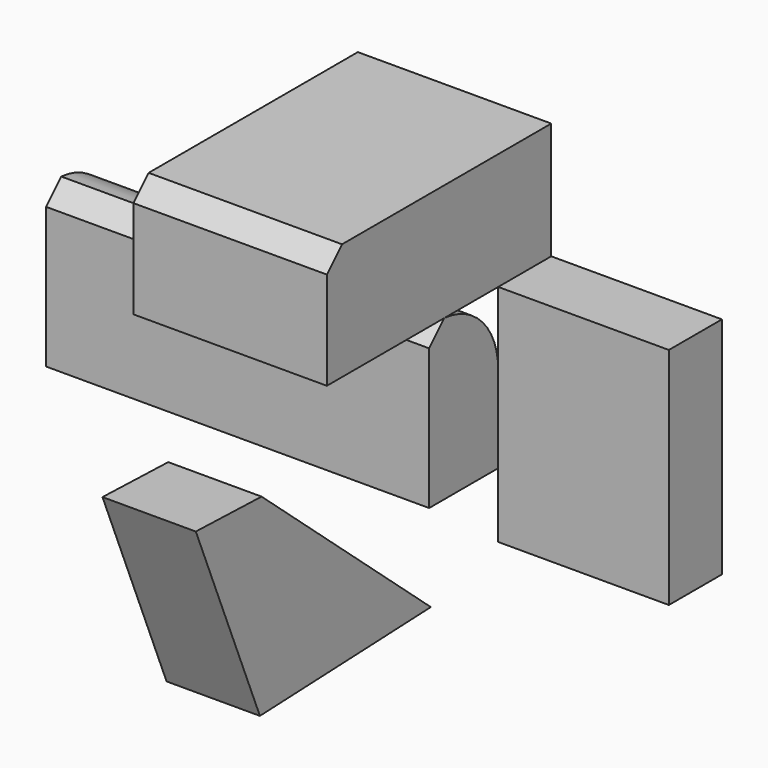
from build123d import *

# Parameters (mm, degrees)
F0_W        = 23.1258124113
F0_H        = 42.7482295781
F1_DEPTH    = 102.616
F2_DEPTH    = 51.816
F3_DEPTH    = 45.72
F4_SIZE     = 5.08
F4_2_SIZE   = 5.08
F5_T1_DEPTH = 200.4123170871
F7_DEPTH    = 12.5


# Not quite as in the source:
# - a fillet or chamfer that OpenCascade refuses, or shapes differently, is made with other operations: its cross-section is extruded or revolved along the edge and cut away or added
# - a feature of the source that left no trace in its solid (it failed there, or was rolled back) is left out


with BuildPart() as f1:
    # F0 (on Right) → F1 (new body)
    with BuildSketch(Plane.YZ):
        with Locations((59.9930435419, 8.5665853694)):
            Rectangle(F0_W, F0_H)
    extrude(amount=-F1_DEPTH)

    # F4
    f4_edges = [f1.edges().sort_by_distance(p)[0] for p in [
        (-51.308, 48.430137, 29.9407),
    ]]
    chamfer(f4_edges, length=F4_SIZE)

    # F5: fillet of radius 19.622727835 on 1 edges, made by hand

    # F5_s2 → F5_t1 (cut)
    with BuildSketch(Plane.YZ.offset(-151.5141585435)):
        with BuildLine():
            ThreePointArc((53.5101373363, 29.9407001585), (66.355337393, 23.687601957), (71.5559497476, 10.3814367411))
            Line((71.5559497476, 10.3814367411), (71.5559497476, 29.9407001585))
            Line((71.5559497476, 29.9407001585), (53.5101373363, 29.9407001585))
        make_face()
    extrude(amount=F5_T1_DEPTH, mode=Mode.SUBTRACT)


with BuildPart() as f2:
    # F0 (on Right) → F2 (new body)
    with BuildSketch(Plane.YZ):
        Polygon((89.3192514777, 29.9407001585), (89.3192514777, 61.2500272691), (14.1880903393, 61.2500272691), (14.1880903393, 29.9407001585), (48.4301373363, 29.9407001585), (71.5559497476, 29.9407001585), align=None)
    extrude(amount=-F2_DEPTH)

    # F4#2
    f4_2_edges = [f2.edges().sort_by_distance(p)[0] for p in [
        (-25.908, 14.18809, 61.250027),
    ]]
    chamfer(f4_2_edges, length=F4_2_SIZE)


with BuildPart() as f3:
    # F0 (on Right) → F3 (new body)
    with BuildSketch(Plane.YZ):
        Polygon((89.3192514777, -30.2083920687), (89.3192514777, 29.9407001585), (71.5559497476, 29.9407001585), (71.5559497476, -12.8075294197), (71.5559497476, -30.2083920687), align=None)
    extrude(amount=F3_DEPTH)


with BuildPart() as f7:
    # F0 (on Right) → F7 (new body, symmetric)
    with BuildSketch(Plane.YZ):
        Polygon((33.377405256, -25.9779412299), (-23.3115255833, 23.1231357902), (-45.3274697065, 23.8340292126), (-23.8601844758, -28.3768214285), align=None)
    extrude(amount=F7_DEPTH, both=True)


solid = Compound([f1.part, f2.part, f3.part, f7.part])
